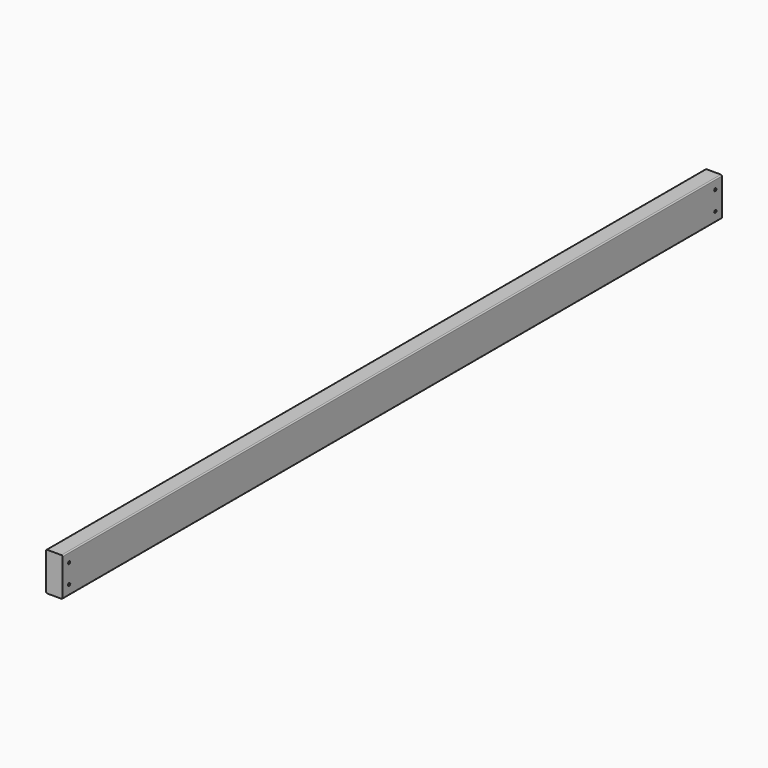
from build123d import *

# Parameters (mm, degrees)
F0_W          = 38.1
F0_H          = 88.9
F1_DEPTH      = 952.5
F1_DEPTH_BACK = 952.5
F2_R          = 3.175
F3_DEPTH      = 12.7
F4_R          = 2.54


# Not quite as in the source:
# - a length typed as a fraction of an inch, garbled in the dataset ("3 / 203.2 mm" for 3/8 in), is restored
# - a pattern or mirror of a feature is missing from the dataset's text; its kind, count and spacing are read off the source's solid


with BuildPart() as f1:
    # F0 (on Front) → F1 (new body, two sides)
    with BuildSketch(Plane.XZ) as f1_sk:
        Rectangle(F0_W, F0_H)
    extrude(amount=F1_DEPTH)
    extrude(f1_sk.sketch, amount=-F1_DEPTH_BACK)

    # F2 (on face) → F3 (cut)
    with BuildSketch(Plane.YZ.offset(19.05)):
        with Locations((-933.45, 22.225)):
            Circle(F2_R)
    f3 = extrude(amount=-F3_DEPTH, mode=Mode.SUBTRACT)

    # F3_copies: F3 across plane
    add(f3.mirror(Plane(origin=(0, 0, 0), x_dir=(0, 0.0238027779, 0.9997166737), z_dir=(0, 0.9997166737, -0.0238027779))), mode=Mode.SUBTRACT)

    # F3_copies1: F3 across plane
    add(f3.mirror(Plane(origin=(0, 0, 0), x_dir=(-1, 0, 0), z_dir=(0, 0, -1))), mode=Mode.SUBTRACT)

    # F3_copies2: F3 across plane
    add(f3.mirror(Plane.ZX), mode=Mode.SUBTRACT)

    # F4
    f4_edges = [f1.edges().sort_by_distance(p)[0] for p in [
        (19.05, 0, 44.45),
        (-19.05, 0, 44.45),
        (19.05, 0, -44.45),
        (-19.05, 0, -44.45),
    ]]
    fillet(f4_edges, radius=F4_R)


solid = f1.part
